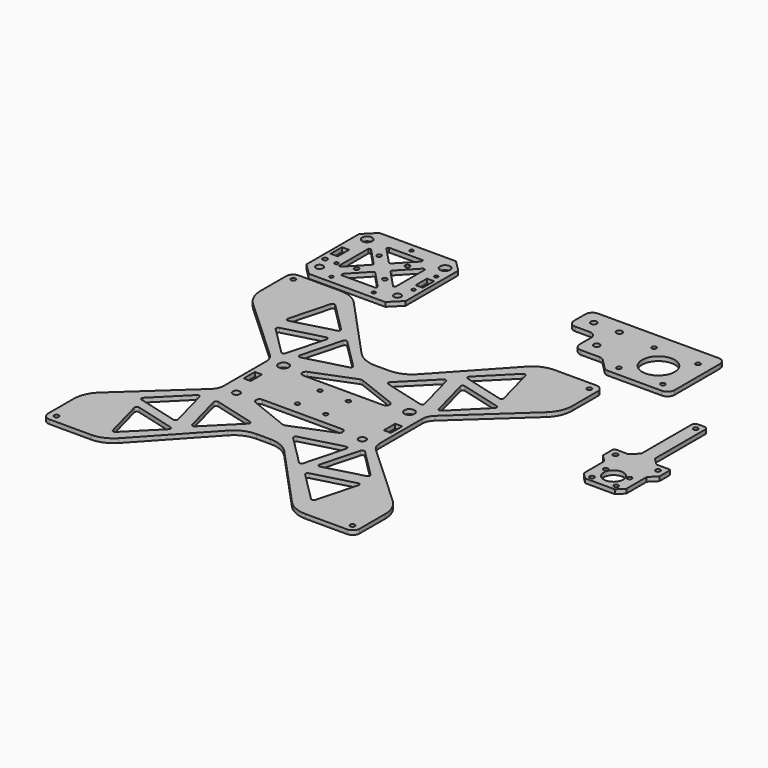
from build123d import *

# Parameters (mm, degrees)
F0_R     = 1.2573
F0_R_2   = 2.55
F0_R_3   = 1.6
F0_R_4   = 1.25
F0_W     = 5
F0_H     = 10
F0_R_5   = 3.556
F1_DEPTH = 3
F0_R_6   = 1.65
F0_R_7   = 1.525
F0_R_8   = 3.555
F0_R_9   = 2.1
F0_R_10  = 11.5
F0_R_11  = 1.5881
F0_R_12  = 6.877
F0_R_13  = 1.6383


# Not quite as in the source:
# - ends of sketch curves that miss each other by under 0.0002 mm in the source are joined


with BuildPart() as f1:
    # F0 (on Top) → F1 (new body)
    with BuildSketch(Plane.XY):
        Polygon((-197.403842, 81.066687), (-143.403842, 81.066687), (-135.403842, 89.066687), (-135.403842, 135.447257), (-143.403842, 143.447257), (-197.403842, 143.447257), (-205.403842, 135.447257), (-205.403842, 89.066687), align=None)
        with Locations((-185.433699, 86.03683)):
            Circle(F0_R, mode=Mode.SUBTRACT)
        with Locations((-155.488942, 86.03683)):
            Circle(F0_R, mode=Mode.SUBTRACT)
        with Locations((-197.903842, 91.251172)):
            Circle(F0_R_2, mode=Mode.SUBTRACT)
        with Locations((-201.358869, 100.41183)):
            Circle(F0_R_3, mode=Mode.SUBTRACT)
        with Locations((-193.358869, 100.41183)):
            Circle(F0_R_4, mode=Mode.SUBTRACT)
        with Locations((-180.63241, 102.256972)):
            Circle(F0_R_3, mode=Mode.SUBTRACT)
        with BuildLine():
            ThreePointArc((-171.3271483155, 104.852883298), (-170.4038416567, 105.250871), (-169.4805352131, 104.8528827988))
            Line((-169.4805352131, 104.8528827988), (-157.777089, 92.460998))
            Line((-157.777089, 92.460998), (-158.403842, 91.006972))
            Line((-158.403842, 91.006972), (-182.403842, 91.006972))
            Line((-182.403842, 91.006972), (-183.030595, 92.460998))
            Line((-183.030595, 92.460998), (-171.3271483155, 104.852883298))
        make_face(mode=Mode.SUBTRACT)
        with Locations((-160.63241, 102.256972)):
            Circle(F0_R_3, mode=Mode.SUBTRACT)
        with Locations((-142.903842, 91.251172)):
            Circle(F0_R_2, mode=Mode.SUBTRACT)
        with Locations((-140.403842, 102.256972)):
            Circle(F0_R_4, mode=Mode.SUBTRACT)
        with Locations((-200.403842, 112.256972)):
            Rectangle(F0_W, F0_H, mode=Mode.SUBTRACT)
        with BuildLine():
            ThreePointArc((-177.0607422131, 112.8789837988), (-176.714049, 112.006972), (-177.0607422131, 111.1349602012))
            Line((-177.0607422131, 111.1349602012), (-189.030595, 98.460998))
            Line((-189.030595, 98.460998), (-190.403842, 99.006972))
            Line((-190.403842, 99.006972), (-190.403842, 125.006973))
            Line((-190.403842, 125.006973), (-189.030595, 125.552946))
            Line((-189.030595, 125.552946), (-177.0607422131, 112.8789837988))
        make_face(mode=Mode.SUBTRACT)
        with Locations((-180.63241, 122.256972)):
            Circle(F0_R_3, mode=Mode.SUBTRACT)
        with BuildLine():
            Line((-150.403842, 125.006973), (-150.403842, 99.006972))
            Line((-150.403842, 99.006972), (-151.777089, 98.460998))
            Line((-151.777089, 98.460998), (-163.746942, 111.13496))
            ThreePointArc((-163.746942, 111.13496), (-164.093635, 112.006972), (-163.7469417869, 112.8789837988))
            Line((-163.7469417869, 112.8789837988), (-151.777089, 125.552946))
            Line((-151.777089, 125.552946), (-150.403842, 125.006973))
        make_face(mode=Mode.SUBTRACT)
        with BuildLine():
            Line((-157.777089, 131.552946), (-169.480535, 119.161062))
            ThreePointArc((-169.480535, 119.161062), (-170.4038416567, 118.763074), (-171.3271483155, 119.161061702))
            Line((-171.3271483155, 119.161061702), (-183.030595, 131.552946))
            Line((-183.030595, 131.552946), (-182.403842, 133.006973))
            Line((-182.403842, 133.006973), (-158.403842, 133.006973))
            Line((-158.403842, 133.006973), (-157.777089, 131.552946))
        make_face(mode=Mode.SUBTRACT)
        with Locations((-160.63241, 122.256972)):
            Circle(F0_R_3, mode=Mode.SUBTRACT)
        with Locations((-197.903842, 133.262772)):
            Circle(F0_R_5, mode=Mode.SUBTRACT)
        with Locations((-170.403842, 138.022483)):
            Circle(F0_R, mode=Mode.SUBTRACT)
        with Locations((-140.403842, 112.256972)):
            Rectangle(F0_W, F0_H, mode=Mode.SUBTRACT)
        with Locations((-140.403842, 122.256972)):
            Circle(F0_R_4, mode=Mode.SUBTRACT)
        with Locations((-142.903842, 133.262772)):
            Circle(F0_R_5, mode=Mode.SUBTRACT)
    extrude(amount=F1_DEPTH)


with BuildPart() as f1b:
    # F0 (on Top) → F1, piece 2 (new body)
    with BuildSketch(Plane.XY):
        with BuildLine():
            ThreePointArc((8.1515359496, 33.8712540546), (12.9142850739, 40.5489136613), (14.596158, 48.576754))
            Line((14.596158, 48.576754), (14.596158, 71.066687))
            ThreePointArc((14.596158, 71.066687), (13.1316919059, 74.6022209059), (9.596158, 76.066687))
            Line((9.596158, 76.066687), (-19.693952, 76.066687))
            ThreePointArc((-19.693952, 76.066687), (-27.7217923387, 74.3848140739), (-34.3994519454, 69.6220649496))
            Line((-34.3994519454, 69.6220649496), (-75.636411, 24.886309))
            ThreePointArc((-75.636411, 24.886309), (-82.3140699717, 20.1235597901), (-90.34191, 18.441687))
            Line((-90.34191, 18.441687), (-100.465774, 18.441687))
            ThreePointArc((-100.465774, 18.441687), (-108.4936140283, 20.1235597901), (-115.171273486, 24.886308552))
            Line((-115.171273486, 24.886308552), (-156.408232, 69.622065))
            ThreePointArc((-156.408232, 69.622065), (-163.0858916613, 74.3848140739), (-171.113732, 76.066687))
            Line((-171.113732, 76.066687), (-200.403842, 76.066687))
            ThreePointArc((-200.403842, 76.066687), (-203.9393759059, 74.6022209059), (-205.403842, 71.066687))
            Line((-205.403842, 71.066687), (-205.403842, 48.576754))
            ThreePointArc((-205.403842, 48.576754), (-203.7219690739, 40.5489136613), (-198.9592199496, 33.8712540546))
            Line((-198.9592199496, 33.8712540546), (-153.626129, -7.916321))
            ThreePointArc((-153.626129, -7.916321), (-151.244754463, -11.2551508306), (-150.403818, -15.269071))
            Line((-150.403818, -15.269071), (-150.403818, -52.597555))
            ThreePointArc((-150.403818, -52.597555), (-151.244754327, -56.611474859), (-153.6261285268, -59.9503045133))
            Line((-153.6261285268, -59.9503045133), (-198.95922, -101.73788))
            ThreePointArc((-198.95922, -101.73788), (-203.7219690739, -108.4155396613), (-205.403842, -116.44338))
            Line((-205.403842, -116.44338), (-205.403842, -138.933313))
            ThreePointArc((-205.403842, -138.933313), (-203.9393759059, -142.4688469059), (-200.403842, -143.933313))
            Line((-200.403842, -143.933313), (-171.113732, -143.933313))
            ThreePointArc((-171.113732, -143.933313), (-163.0858916613, -142.2514400739), (-156.4082320546, -137.4886909496))
            Line((-156.4082320546, -137.4886909496), (-115.171273, -92.752935))
            ThreePointArc((-115.171273, -92.752935), (-108.4936140283, -87.9901857901), (-100.465774, -86.308313))
            Line((-100.465774, -86.308313), (-90.34191, -86.308313))
            ThreePointArc((-90.34191, -86.308313), (-82.3140696613, -87.9901859261), (-75.6364100546, -92.7529350504))
            Line((-75.6364100546, -92.7529350504), (-34.399452, -137.488691))
            ThreePointArc((-34.399452, -137.488691), (-27.7217923387, -142.2514400739), (-19.693952, -143.933313))
            Line((-19.693952, -143.933313), (9.596158, -143.933313))
            ThreePointArc((9.596158, -143.933313), (13.1316919059, -142.4688469059), (14.596158, -138.933313))
            Line((14.596158, -138.933313), (14.596158, -116.44338))
            ThreePointArc((14.596158, -116.44338), (12.9142850739, -108.4155396613), (8.1515359496, -101.7378800546))
            Line((8.1515359496, -101.7378800546), (-37.181555, -59.950304))
            ThreePointArc((-37.181555, -59.950304), (-39.562929673, -56.611474859), (-40.403866, -52.597555))
            Line((-40.403866, -52.597555), (-40.403866, -15.269071))
            ThreePointArc((-40.403866, -15.269071), (-39.562929537, -11.2551508306), (-37.1815549748, -7.9163210273))
            Line((-37.1815549748, -7.9163210273), (8.1515359496, 33.8712540546))
        make_face()
        with Locations((-199.903842, -138.433313)):
            Circle(F0_R_6, mode=Mode.SUBTRACT)
        with BuildLine():
            ThreePointArc((-172.6950168988, -103.7169259729), (-172.3067881718, -102.2680378282), (-170.8579000271, -101.8798091012))
            Line((-170.8579000271, -101.8798091012), (-142.416345, -109.500701))
            ThreePointArc((-142.416345, -109.500701), (-141.3556851818, -110.5613607265), (-141.7439138282, -112.0102491718))
            Line((-141.7439138282, -112.0102491718), (-162.564576, -132.830912))
            ThreePointArc((-162.564576, -132.830912), (-164.013464932, -133.2191409097), (-165.0741255818, -132.1584811559))
            Line((-165.0741255818, -132.1584811559), (-172.6950168988, -103.7169259729))
        make_face(mode=Mode.SUBTRACT)
        with BuildLine():
            ThreePointArc((-145.0741251012, -99.6584810271), (-145.4623541697, -101.1073695133), (-146.9112429059, -101.4955976488))
            Line((-146.9112429059, -101.4955976488), (-175.352797, -93.874707))
            ThreePointArc((-175.352797, -93.874707), (-176.4134566932, -92.81404674), (-176.0252286718, -91.3651583282))
            Line((-176.0252286718, -91.3651583282), (-155.204566, -70.544495))
            ThreePointArc((-155.204566, -70.544495), (-153.7556776015, -70.1562662153), (-152.6950173512, -71.2169260941))
            Line((-152.6950173512, -71.2169260941), (-145.0741251012, -99.6584810271))
        make_face(mode=Mode.SUBTRACT)
        with BuildLine():
            ThreePointArc((-112.4163448441, -77.0007004182), (-111.3556851818, -78.0613607265), (-111.7439138282, -79.5102491718))
            Line((-111.7439138282, -79.5102491718), (-132.564576, -100.330912))
            ThreePointArc((-132.564576, -100.330912), (-134.013464932, -100.7191409097), (-135.0741255818, -99.6584811559))
            Line((-135.0741255818, -99.6584811559), (-142.695017, -71.216926))
            ThreePointArc((-142.695017, -71.216926), (-142.3067881718, -69.7680378282), (-140.8579000271, -69.3798091012))
            Line((-140.8579000271, -69.3798091012), (-112.4163448441, -77.0007004182))
        make_face(mode=Mode.SUBTRACT)
        with BuildLine():
            ThreePointArc((-49.2828821718, -107.2628011718), (-49.6711107847, -105.8139126015), (-48.6104509059, -104.7532523512))
            Line((-48.6104509059, -104.7532523512), (-20.168896, -97.13236))
            ThreePointArc((-20.168896, -97.13236), (-18.7200074867, -97.5205891697), (-18.3317793512, -98.9694779059))
            Line((-18.3317793512, -98.9694779059), (-25.952671, -127.411032))
            ThreePointArc((-25.952671, -127.411032), (-27.0133307265, -128.4716918182), (-28.4622191718, -128.0834631718))
            Line((-28.4622191718, -128.0834631718), (-49.2828821718, -107.2628011718))
        make_face(mode=Mode.SUBTRACT)
        with BuildLine():
            ThreePointArc((-52.6688959729, -67.1323601012), (-51.2200074867, -67.5205891697), (-50.8317793512, -68.9694779059))
            Line((-50.8317793512, -68.9694779059), (-58.452671, -97.411032))
            ThreePointArc((-58.452671, -97.411032), (-59.5133307265, -98.4716918182), (-60.9622191718, -98.0834631718))
            Line((-60.9622191718, -98.0834631718), (-81.782882, -77.262801))
            ThreePointArc((-81.782882, -77.262801), (-82.1711107847, -75.8139126015), (-81.1104509059, -74.7532523512))
            Line((-81.1104509059, -74.7532523512), (-52.6688959729, -67.1323601012))
        make_face(mode=Mode.SUBTRACT)
        with BuildLine():
            ThreePointArc((-48.6104510271, -94.7532518988), (-50.0593391718, -94.3650231718), (-50.4475678988, -92.9161350271))
            Line((-50.4475678988, -92.9161350271), (-43.206227, -65.891081))
            ThreePointArc((-43.206227, -65.891081), (-42.1455663985, -64.8304212153), (-40.6966778282, -65.2186498282))
            Line((-40.6966778282, -65.2186498282), (-20.912966, -85.002362))
            ThreePointArc((-20.912966, -85.002362), (-20.5247372153, -86.4512503985), (-21.5853970941, -87.5119106488))
            Line((-21.5853970941, -87.5119106488), (-48.6104510271, -94.7532518988))
        make_face(mode=Mode.SUBTRACT)
        with Locations((-139.848818, -54.741065)):
            Circle(F0_R_2, mode=Mode.SUBTRACT)
        with Locations((-105.403842, -43.933313)):
            Circle(F0_R_7, mode=Mode.SUBTRACT)
        with Locations((-144.903818, -33.933313)):
            Rectangle(F0_W, F0_H, mode=Mode.SUBTRACT)
        with Locations((-105.403842, -23.933313)):
            Circle(F0_R_7, mode=Mode.SUBTRACT)
        with Locations((-139.848818, -13.122495)):
            Circle(F0_R_8, mode=Mode.SUBTRACT)
        with BuildLine():
            ThreePointArc((-124.4475411847, -57.0984444605), (-125.9957610067, -54.2594758751), (-123.501834, -52.201065))
            Line((-123.501834, -52.201065), (-67.284508, -52.201065))
            ThreePointArc((-67.284508, -52.201065), (-64.7908847365, -54.2579055855), (-66.335832759, -57.0972515985))
            Line((-66.335832759, -57.0972515985), (-94.393347, -68.394091))
            ThreePointArc((-94.393347, -68.394091), (-95.3404230681, -68.5779034967), (-96.2877297006, -68.3952832536))
            Line((-96.2877297006, -68.3952832536), (-124.4475411847, -57.0984444605))
        make_face(mode=Mode.SUBTRACT)
        with Locations((-85.403842, -43.933313)):
            Circle(F0_R_7, mode=Mode.SUBTRACT)
        with Locations((-50.958866, -54.741065)):
            Circle(F0_R_2, mode=Mode.SUBTRACT)
        with Locations((-85.403842, -23.933313)):
            Circle(F0_R_7, mode=Mode.SUBTRACT)
        with BuildLine():
            ThreePointArc((-96.6323712726, 0.3553006936), (-95.703217, 0.531348), (-94.7740627274, 0.3553006936))
            Line((-94.7740627274, 0.3553006936), (-66.498233, -10.758542))
            ThreePointArc((-66.498233, -10.758542), (-64.9317868536, -13.5953373724), (-67.427387, -15.662495))
            Line((-67.427387, -15.662495), (-123.979047, -15.662495))
            ThreePointArc((-123.979047, -15.662495), (-126.4746471464, -13.5953373724), (-124.9082009322, -10.7585421726))
            Line((-124.9082009322, -10.7585421726), (-96.6323712726, 0.3553006936))
        make_face(mode=Mode.SUBTRACT)
        with Locations((-45.903866, -33.933313)):
            Rectangle(F0_W, F0_H, mode=Mode.SUBTRACT)
        with Locations((-50.958866, -13.122495)):
            Circle(F0_R_8, mode=Mode.SUBTRACT)
        with Locations((9.096158, -138.433313)):
            Circle(F0_R_6, mode=Mode.SUBTRACT)
        with BuildLine():
            ThreePointArc((-142.6688959729, 27.8676398988), (-141.2200074867, 27.4794108303), (-140.8317793512, 26.0305220941))
            Line((-140.8317793512, 26.0305220941), (-148.07312, -0.994531))
            ThreePointArc((-148.07312, -0.994531), (-149.13378026, -2.0551906932), (-150.5826686718, -1.6669626718))
            Line((-150.5826686718, -1.6669626718), (-170.366381, 18.116749))
            ThreePointArc((-170.366381, 18.116749), (-170.7546099097, 19.565637932), (-169.6939501559, 20.6262985818))
            Line((-169.6939501559, 20.6262985818), (-142.6688959729, 27.8676398988))
        make_face(mode=Mode.SUBTRACT)
        with BuildLine():
            ThreePointArc((-138.6104510271, 0.2467481012), (-140.0593391718, 0.6349768282), (-140.4475678988, 2.0838649729))
            Line((-140.4475678988, 2.0838649729), (-132.826677, 30.52542))
            ThreePointArc((-132.826677, 30.52542), (-131.7660163985, 31.5860797847), (-130.3171278282, 31.1978511718))
            Line((-130.3171278282, 31.1978511718), (-109.496465, 10.377189))
            ThreePointArc((-109.496465, 10.377189), (-109.1082360903, 8.928300068), (-110.1688958441, 7.8676394182))
            Line((-110.1688958441, 7.8676394182), (-138.6104510271, 0.2467481012))
        make_face(mode=Mode.SUBTRACT)
        with BuildLine():
            ThreePointArc((-141.9964653282, 40.3771886718), (-141.6082360903, 38.928300068), (-142.6688958441, 37.8676394182))
            Line((-142.6688958441, 37.8676394182), (-171.110451, 30.246748))
            ThreePointArc((-171.110451, 30.246748), (-172.5593391718, 30.6349768282), (-172.9475678988, 32.0838649729))
            Line((-172.9475678988, 32.0838649729), (-165.326677, 60.52542))
            ThreePointArc((-165.326677, 60.52542), (-164.2660163985, 61.5860797847), (-162.8171278282, 61.1978511718))
            Line((-162.8171278282, 61.1978511718), (-141.9964653282, 40.3771886718))
        make_face(mode=Mode.SUBTRACT)
        with Locations((-199.903842, 70.566687)):
            Circle(F0_R_6, mode=Mode.SUBTRACT)
        with BuildLine():
            ThreePointArc((-60.7096676718, 28.9504026718), (-59.26077926, 29.3386306932), (-58.2001193512, 28.2779709059))
            Line((-58.2001193512, 28.2779709059), (-50.579228, -0.163583))
            ThreePointArc((-50.579228, -0.163583), (-50.9674564867, -1.6124718303), (-52.4163449729, -2.0007008988))
            Line((-52.4163449729, -2.0007008988), (-80.8579, 5.620191))
            ThreePointArc((-80.8579, 5.620191), (-81.9185597847, 6.6808516015), (-81.5303311718, 8.1297401718))
            Line((-81.5303311718, 8.1297401718), (-60.7096676718, 28.9504026718))
        make_face(mode=Mode.SUBTRACT)
        with BuildLine():
            ThreePointArc((-48.2001195818, 28.2779708441), (-47.8118911718, 29.7268601718), (-46.3630018441, 30.1150885818))
            Line((-46.3630018441, 30.1150885818), (-17.921448, 22.494197))
            ThreePointArc((-17.921448, 22.494197), (-16.8607873403, 21.433536865), (-17.2490158282, 19.9846478282))
            Line((-17.2490158282, 19.9846478282), (-38.069679, -0.836015))
            ThreePointArc((-38.069679, -0.836015), (-39.518567865, -1.2242436597), (-40.5792278988, -0.1635829729))
            Line((-40.5792278988, -0.1635829729), (-48.2001195818, 28.2779708441))
        make_face(mode=Mode.SUBTRACT)
        with BuildLine():
            ThreePointArc((-20.5792283512, 32.3364169059), (-20.9674564867, 30.8875281697), (-22.4163449729, 30.4992991012))
            Line((-22.4163449729, 30.4992991012), (-50.8579, 38.120191))
            ThreePointArc((-50.8579, 38.120191), (-51.9185597847, 39.1808516015), (-51.5303311718, 40.6297401718))
            Line((-51.5303311718, 40.6297401718), (-30.709668, 61.450403))
            ThreePointArc((-30.709668, 61.450403), (-29.26077926, 61.8386306932), (-28.2001193512, 60.7779709059))
            Line((-28.2001193512, 60.7779709059), (-20.5792283512, 32.3364169059))
        make_face(mode=Mode.SUBTRACT)
        with Locations((9.096158, 70.566687)):
            Circle(F0_R_6, mode=Mode.SUBTRACT)
    extrude(amount=F1_DEPTH)


with BuildPart() as f1c:
    # F0 (on Top) → F1, piece 3 (new body)
    with BuildSketch(Plane.XY):
        with BuildLine():
            ThreePointArc((41.793117, 93.613331), (45.3286509059, 95.0777970941), (46.793117, 98.613331))
            Line((46.793117, 98.613331), (46.793117, 138.613331))
            ThreePointArc((46.793117, 138.613331), (45.3286509059, 142.1488649059), (41.793117, 143.613331))
            Line((41.793117, 143.613331), (-43.206883, 143.613331))
            ThreePointArc((-43.206883, 143.613331), (-46.7424169059, 142.1488649059), (-48.206883, 138.613331))
            Line((-48.206883, 138.613331), (-48.206883, 128.613331))
            ThreePointArc((-48.206883, 128.613331), (-46.7424169059, 125.0777970941), (-43.206883, 123.613331))
            Line((-43.206883, 123.613331), (-33.206883, 123.613331))
            ThreePointArc((-33.206883, 123.613331), (-29.6713490941, 122.1488649059), (-28.206883, 118.613331))
            Line((-28.206883, 118.613331), (-28.206883, 108.613331))
            ThreePointArc((-28.206883, 108.613331), (-26.7424169059, 105.0777970941), (-23.206883, 103.613331))
            Line((-23.206883, 103.613331), (-10.277951, 103.613331))
            ThreePointArc((-10.277951, 103.613331), (-8.3645338382, 103.2327286626), (-6.7424170941, 102.1488649059))
            Line((-6.7424170941, 102.1488649059), (0.328651, 95.077797))
            ThreePointArc((0.328651, 95.077797), (1.9507671648, 93.9939332021), (3.864184, 93.613331))
            Line((3.864184, 93.613331), (41.793117, 93.613331))
        make_face()
        with Locations((-20.206883, 113.613331)):
            Circle(F0_R_9, mode=Mode.SUBTRACT)
        with Locations((-38.206883, 133.613331)):
            Circle(F0_R_9, mode=Mode.SUBTRACT)
        with Locations((-20.206883, 133.613331)):
            Circle(F0_R_9, mode=Mode.SUBTRACT)
        with Locations((6.293117, 100.113331)):
            Circle(F0_R_3, mode=Mode.SUBTRACT)
        with Locations((37.293117, 100.113331)):
            Circle(F0_R_3, mode=Mode.SUBTRACT)
        with Locations((21.793117, 115.613331)):
            Circle(F0_R_10, mode=Mode.SUBTRACT)
        with Locations((6.293117, 131.113331)):
            Circle(F0_R_3, mode=Mode.SUBTRACT)
        with Locations((37.293117, 131.113331)):
            Circle(F0_R_3, mode=Mode.SUBTRACT)
    extrude(amount=F1_DEPTH)


with BuildPart() as f1d:
    # F0 (on Top) → F1, piece 4 (new body)
    with BuildSketch(Plane.XY):
        with BuildLine():
            ThreePointArc((82.386358, 74.750839), (80.5903067758, 74.0068902242), (79.846358, 72.210839))
            Line((79.846358, 72.210839), (79.846358, 28.051041))
            Line((79.846358, 28.051041), (74.766358, 22.971041))
            Line((74.766358, 22.971041), (65.866158, 22.971041))
            ThreePointArc((65.866158, 22.971041), (64.9681323879, 22.5990666121), (64.596158, 21.701041))
            Line((64.596158, 21.701041), (64.596158, 13.030756))
            Line((64.596158, 13.030756), (69.596158, 8.030756))
            Line((69.596158, 8.030756), (69.596158, -9.969244))
            Line((69.596158, -9.969244), (74.096158, -14.469244))
            Line((74.096158, -14.469244), (95.096158, -14.469244))
            Line((95.096158, -14.469244), (99.596158, -9.969244))
            Line((99.596158, -9.969244), (99.596158, 8.030756))
            Line((99.596158, 8.030756), (104.596158, 13.030756))
            Line((104.596158, 13.030756), (104.596158, 21.701041))
            ThreePointArc((104.596158, 21.701041), (104.2241836121, 22.5990666121), (103.326158, 22.971041))
            Line((103.326158, 22.971041), (94.425958, 22.971041))
            Line((94.425958, 22.971041), (89.345958, 28.051041))
            Line((89.345958, 28.051041), (89.345958, 72.210839))
            ThreePointArc((89.345958, 72.210839), (88.6020092242, 74.0068902242), (86.805958, 74.750839))
            Line((86.805958, 74.750839), (82.386358, 74.750839))
        make_face()
        with Locations((76.096158, -10.869244)):
            Circle(F0_R_11, mode=Mode.SUBTRACT)
        with Locations((93.096158, -10.869244)):
            Circle(F0_R_11, mode=Mode.SUBTRACT)
        with Locations((84.596158, -2.469244)):
            Circle(F0_R_12, mode=Mode.SUBTRACT)
        with Locations((76.096158, 1.130756)):
            Circle(F0_R_11, mode=Mode.SUBTRACT)
        with Locations((93.096158, 1.130756)):
            Circle(F0_R_11, mode=Mode.SUBTRACT)
        with Locations((69.5663, 18.000899)):
            Circle(F0_R_13, mode=Mode.SUBTRACT)
        with Locations((99.511058, 18.000899)):
            Circle(F0_R_13, mode=Mode.SUBTRACT)
        with Locations((84.596158, 69.986553)):
            Circle(F0_R_13, mode=Mode.SUBTRACT)
    extrude(amount=F1_DEPTH)


solid = Compound([f1.part, f1b.part, f1c.part, f1d.part])
